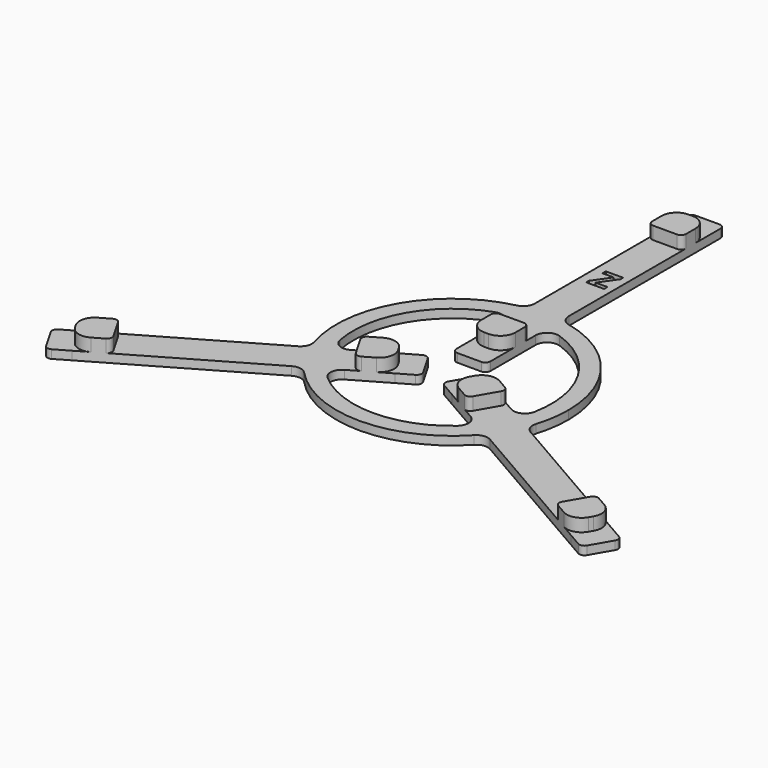
from build123d import *

# Parameters (mm, degrees)
F0_W         = 8
F0_H         = 5
F0_H_2       = 7.5
F1_DEPTH     = 2
F2_DEPTH     = 5
F3_R         = 3.5
F4_TEXT_SIZE = 7.9356185678
F5_DEPTH     = 1
F6_R         = 2.7015952547
F7_R         = 1.2


# Not quite as in the source:
# - Text() gives the source's letters only with a copy of the font that has no kerning and outlines rounded to 1/6400 em; it was checked with that copy


with BuildPart() as f1:
    # F0 (on Top) → F1 (new body)
    with BuildSketch(Plane.XY):
        with BuildLine():
            ThreePointArc((-4, 26.9901612957), (0, 27.2849556857), (4, 26.9901612957))
            Line((4, 26.9901612957), (4, 62.5))
            Line((4, 62.5), (-4, 62.5))
            Line((-4, 62.5), (-4, 26.9901612957))
        make_face()
        with BuildLine():
            ThreePointArc((-4, 22.9388134236), (0, 23.2849556857), (4, 22.9388134236))
            Line((4, 22.9388134236), (4, 26.9901612957))
            ThreePointArc((4, 26.9901612957), (0, 27.2849556857), (-4, 26.9901612957))
            Line((-4, 26.9901612957), (-4, 22.9388134236))
        make_face()
        with BuildLine():
            Line((-4, 17.5), (4, 17.5))
            Line((4, 17.5), (4, 22.9388134236))
            ThreePointArc((4, 22.9388134236), (0, 23.2849556857), (-4, 22.9388134236))
            Line((-4, 22.9388134236), (-4, 17.5))
        make_face()
        with Locations((0, 7.5)):
            Rectangle(F0_W, F0_H)
        with BuildLine():
            Line((4, 26.9901612957), (4, 22.9388134236))
            ThreePointArc((4, 22.9388134236), (17.8231448407, 14.9841472654), (23.2849556857, 0))
            ThreePointArc((23.2849556857, 0), (22.9273698401, -4.0650797655), (21.8655951575, -8.0053050967))
            Line((21.8655951575, -8.0053050967), (25.3741653343, -10.0309790327))
            ThreePointArc((25.3741653343, -10.0309790327), (26.8030015435, -5.105674787), (27.2849556857, 0))
            ThreePointArc((27.2849556857, 0), (20.6592428408, 17.8231448407), (4, 26.9901612957))
        make_face()
        with BuildLine():
            ThreePointArc((-21.8655951575, -8.0053050967), (-20.1653631498, 11.6424778428), (-4, 22.9388134236))
            Line((-4, 22.9388134236), (-4, 26.9901612957))
            ThreePointArc((-4, 26.9901612957), (-23.6294647649, 13.6424778428), (-25.3741653343, -10.0309790327))
            Line((-25.3741653343, -10.0309790327), (-21.8655951575, -8.0053050967))
        make_face()
        with Locations((0, 66.25)):
            Rectangle(F0_W, F0_H_2)
        with Locations((0, 72.5)):
            Rectangle(F0_W, F0_H)
        with BuildLine():
            ThreePointArc((-17.8655951575, -14.9335083269), (-20.1653631498, -11.6424778428), (-21.8655951575, -8.0053050967))
            Line((-21.8655951575, -8.0053050967), (-25.3741653343, -10.0309790327))
            ThreePointArc((-25.3741653343, -10.0309790327), (-23.6294647649, -13.6424778428), (-21.3741653343, -16.959182263))
            Line((-21.3741653343, -16.959182263), (-17.8655951575, -14.9335083269))
        make_face()
        with BuildLine():
            Line((-17.1554445662, -5.2858983849), (-21.8655951575, -8.0053050967))
            ThreePointArc((-21.8655951575, -8.0053050967), (-20.1653631498, -11.6424778428), (-17.8655951575, -14.9335083269))
            Line((-17.8655951575, -14.9335083269), (-13.1554445662, -12.2141016151))
            Line((-13.1554445662, -12.2141016151), (-17.1554445662, -5.2858983849))
        make_face()
        Polygon((-6.3301270189, 0.9641016151), (-10.6602540378, -1.5358983849), (-6.6602540378, -8.4641016151), (-2.3301270189, -5.9641016151), align=None)
        with BuildLine():
            ThreePointArc((-21.3741653343, -16.959182263), (-23.6294647649, -13.6424778428), (-25.3741653343, -10.0309790327))
            Line((-25.3741653343, -10.0309790327), (-56.1265877365, -27.7858983849))
            Line((-56.1265877365, -27.7858983849), (-52.1265877365, -34.7141016151))
            Line((-52.1265877365, -34.7141016151), (-21.3741653343, -16.959182263))
        make_face()
        Polygon((-58.6217782649, -38.4641016151), (-62.6217782649, -31.5358983849), (-66.9519052838, -34.0358983849), (-62.9519052838, -40.9641016151), align=None)
        Polygon((6.6602540378, -8.4641016151), (10.6602540378, -1.5358983849), (6.3301270189, 0.9641016151), (2.3301270189, -5.9641016151), align=None)
        with BuildLine():
            ThreePointArc((17.8655951575, -14.9335083269), (20.1653631498, -11.6424778428), (21.8655951575, -8.0053050967))
            Line((21.8655951575, -8.0053050967), (17.1554445662, -5.2858983849))
            Line((17.1554445662, -5.2858983849), (13.1554445662, -12.2141016151))
            Line((13.1554445662, -12.2141016151), (17.8655951575, -14.9335083269))
        make_face()
        with BuildLine():
            Line((25.3741653343, -10.0309790327), (21.8655951575, -8.0053050967))
            ThreePointArc((21.8655951575, -8.0053050967), (20.1653631498, -11.6424778428), (17.8655951575, -14.9335083269))
            Line((17.8655951575, -14.9335083269), (21.3741653343, -16.959182263))
            ThreePointArc((21.3741653343, -16.959182263), (23.6294647649, -13.6424778428), (25.3741653343, -10.0309790327))
        make_face()
        with BuildLine():
            Line((56.1265877365, -27.7858983849), (25.3741653343, -10.0309790327))
            ThreePointArc((25.3741653343, -10.0309790327), (23.6294647649, -13.6424778428), (21.3741653343, -16.959182263))
            Line((21.3741653343, -16.959182263), (52.1265877365, -34.7141016151))
            Line((52.1265877365, -34.7141016151), (56.1265877365, -27.7858983849))
        make_face()
        Polygon((66.9519052838, -34.0358983849), (62.6217782649, -31.5358983849), (58.6217782649, -38.4641016151), (62.9519052838, -40.9641016151), align=None)
        with BuildLine():
            ThreePointArc((17.8655951575, -14.9335083269), (0, -23.2849556857), (-17.8655951575, -14.9335083269))
            Line((-17.8655951575, -14.9335083269), (-21.3741653343, -16.959182263))
            ThreePointArc((-21.3741653343, -16.959182263), (0, -27.2849556857), (21.3741653343, -16.959182263))
            Line((21.3741653343, -16.959182263), (17.8655951575, -14.9335083269))
        make_face()
        Polygon((62.6217782649, -31.5358983849), (56.1265877365, -27.7858983849), (52.1265877365, -34.7141016151), (58.6217782649, -38.4641016151), align=None)
        Polygon((13.1554445662, -12.2141016151), (17.1554445662, -5.2858983849), (10.6602540378, -1.5358983849), (6.6602540378, -8.4641016151), align=None)
        Polygon((-10.6602540378, -1.5358983849), (-17.1554445662, -5.2858983849), (-13.1554445662, -12.2141016151), (-6.6602540378, -8.4641016151), align=None)
        with Locations((0, 13.75)):
            Rectangle(F0_W, F0_H_2)
        Polygon((-52.1265877365, -34.7141016151), (-56.1265877365, -27.7858983849), (-62.6217782649, -31.5358983849), (-58.6217782649, -38.4641016151), align=None)
    extrude(amount=F1_DEPTH)

    # F0 (on Top) → F2 (join)
    with BuildSketch(Plane.XY):
        Polygon((-10.6602540378, -1.5358983849), (-17.1554445662, -5.2858983849), (-13.1554445662, -12.2141016151), (-6.6602540378, -8.4641016151), align=None)
        Polygon((-52.1265877365, -34.7141016151), (-56.1265877365, -27.7858983849), (-62.6217782649, -31.5358983849), (-58.6217782649, -38.4641016151), align=None)
        with Locations((0, 13.75)):
            Rectangle(F0_W, F0_H_2)
        Polygon((13.1554445662, -12.2141016151), (17.1554445662, -5.2858983849), (10.6602540378, -1.5358983849), (6.6602540378, -8.4641016151), align=None)
        Polygon((62.6217782649, -31.5358983849), (56.1265877365, -27.7858983849), (52.1265877365, -34.7141016151), (58.6217782649, -38.4641016151), align=None)
        with Locations((0, 66.25)):
            Rectangle(F0_W, F0_H_2)
    extrude(amount=F2_DEPTH)

    # F3
    f3_edges = [f1.edges().sort_by_distance(p)[0] for p in [
        (-62.621778, -31.535898, 3.5),
        (-58.621778, -38.464102, 3.5),
        (-6.660254, -8.464102, 3.5),
        (-10.660254, -1.535898, 3.5),
        (4, 10, 3.5),
        (-4, 10, 3.5),
        (10.660254, -1.535898, 3.5),
        (6.660254, -8.464102, 3.5),
        (4, 70, 3.5),
        (-4, 70, 3.5),
        (58.621778, -38.464102, 3.5),
        (62.621778, -31.535898, 3.5),
    ]]
    fillet(f3_edges, radius=F3_R)

    # F4 (on face) → F5 (cut)
    with BuildSketch(Plane.XY.offset(2)):
        with Locations((-2.1017339313, 41.715733707)):
            Text('Z', F4_TEXT_SIZE, font='Open Sans', font_style=FontStyle.BOLD, text_align=(TextAlign.LEFT, TextAlign.BOTTOM))
    extrude(amount=-F5_DEPTH, mode=Mode.SUBTRACT)

    # F6
    f6_edges = [f1.edges().sort_by_distance(p)[0] for p in [
        (-4, 22.938813, 1),
        (-21.374165, -16.959182, 1),
        (21.374165, -16.959182, 1),
        (25.374165, -10.030979, 1),
        (4, 26.990161, 1),
        (4, 22.938813, 1),
        (-17.865595, -14.933508, 1),
        (-4, 26.990161, 1),
        (-25.374165, -10.030979, 1),
        (-21.865595, -8.005305, 1),
        (17.865595, -14.933508, 1),
        (21.865595, -8.005305, 1),
    ]]
    fillet(f6_edges, radius=F6_R)

    # F7
    f7_edges = [f1.edges().sort_by_distance(p)[0] for p in [
        (-62.951905, -40.964102, 1),
        (-66.951905, -34.035898, 1),
        (62.951905, -40.964102, 1),
        (66.951905, -34.035898, 1),
        (-4, 75, 1),
        (4, 75, 1),
        (2.330127, -5.964102, 1),
        (6.330127, 0.964102, 1),
        (-4, 5, 1),
        (4, 5, 1),
        (-2.330127, -5.964102, 1),
        (-6.330127, 0.964102, 1),
        (-52.126588, -34.714102, 3.5),
        (-56.126588, -27.785898, 3.5),
        (13.155445, -12.214102, 3.5),
        (4, 17.5, 3.5),
        (-4, 17.5, 3.5),
        (17.155445, -5.285898, 3.5),
        (56.126588, -27.785898, 3.5),
        (52.126588, -34.714102, 3.5),
        (4, 62.5, 3.5),
        (-4, 62.5, 3.5),
        (-13.155445, -12.214102, 3.5),
        (-17.155445, -5.285898, 3.5),
    ]]
    fillet(f7_edges, radius=F7_R)


solid = f1.part
